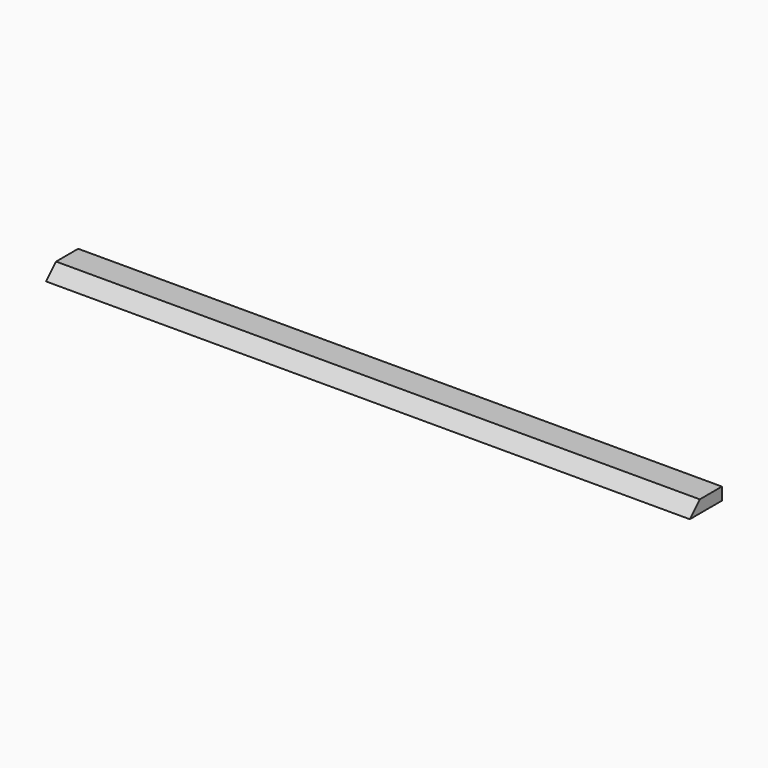
from build123d import *

# Parameters (mm, degrees)
F0_W     = 930
F0_H     = 58
F1_DEPTH = 18
F2_SIZE  = 17.99999


# Not quite as in the source:
# - a fillet or chamfer is up to 0.001 mm smaller than in the source, because OpenCascade refuses the exact size


with BuildPart() as f1:
    # F0 (on Top) → F1 (new body)
    with BuildSketch(Plane.XY):
        Rectangle(F0_W, F0_H)
    extrude(amount=F1_DEPTH)

    # F2 (size 18 in the source; OpenCascade refuses exactly that, so slightly less here)
    f2_edges = [f1.edges().sort_by_distance(p)[0] for p in [
        (0, -29, 18),
    ]]
    chamfer(f2_edges, length=F2_SIZE)


solid = f1.part
